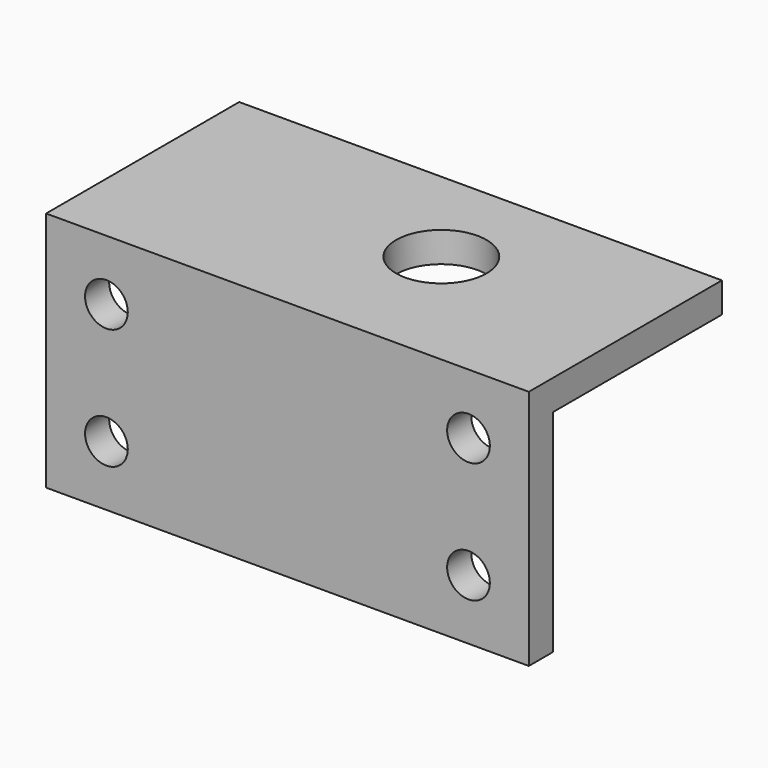
from build123d import *

# Parameters (mm, degrees)
F1_DEPTH = 50.8
F4_D     = 4.4958
F5_D     = 9.525


# Not quite as in the source:
# - a length typed as a fraction of an inch, garbled in the dataset ("3 / 203.2 mm" for 3/8 in), is restored


with BuildPart() as f1:
    # F0 (on Right) → F1 (new body)
    with BuildSketch(Plane.YZ):
        Polygon((0, 25.4), (0, 0), (3.175, 0), (3.175, 22.225), (25.4, 22.225), (25.4, 25.4), align=None)
    extrude(amount=F1_DEPTH)

    # F4 (through all)
    with Locations(Plane(origin=(0, 3.175, 0), x_dir=(-1, 0, 0), z_dir=(0, 1, 0))):
        with Locations((-44.45, 6.35), (-44.45, 19.05), (-6.35, 19.05), (-6.35, 6.35)):
            Hole(F4_D / 2)

    # F5 (through all)
    with Locations(Plane.XY.offset(25.4)):
        with Locations((30.1625, 14.2875)):
            Hole(F5_D / 2)


solid = f1.part
